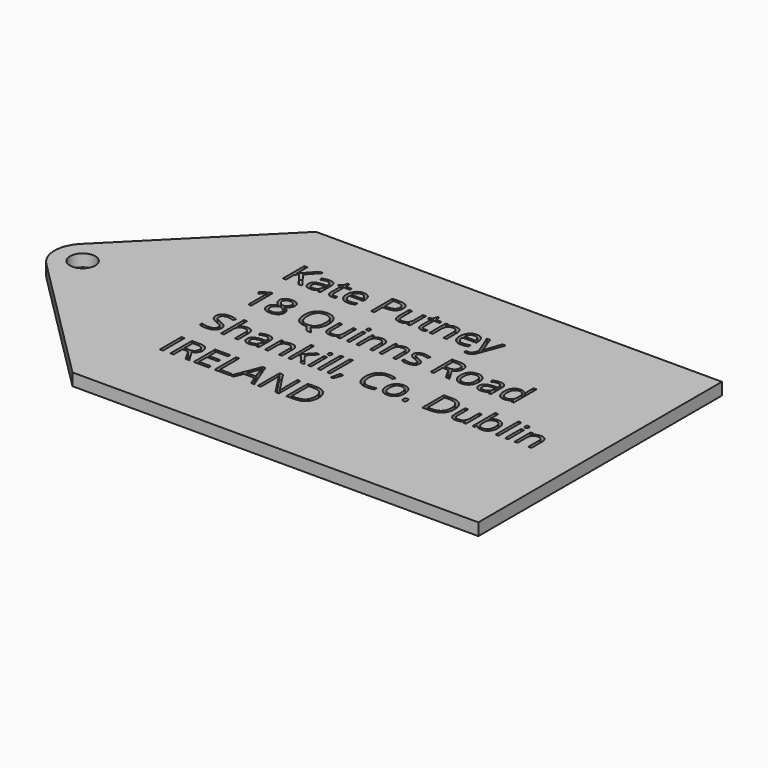
from build123d import *

# Parameters (mm, degrees)
F0_R         = 2.5
F0_W         = 80
F0_H         = 60
F1_DEPTH     = 2.4
F2_TEXT_SIZE = 7.4209044227
F3_DEPTH     = 1.2


# Not quite as in the source:
# - Text() gives the source's letters only with a copy of the font that has no kerning and outlines rounded to 1/6400 em; it was checked with that copy


with BuildPart() as f1:
    # F0 (on Top) → F1 (new body)
    with BuildSketch(Plane.XY):
        with BuildLine():
            Line((-23.865801543, -30), (-23.865801543, 30))
            Line((-23.865801543, 30), (-49.6231608559, 4.2426406871))
            ThreePointArc((-49.6231608559, 4.2426406871), (-51.3805201688, 0), (-49.6231608559, -4.2426406871))
            Line((-49.6231608559, -4.2426406871), (-23.865801543, -30))
        make_face()
        with Locations((-45.865801543, 0)):
            Circle(F0_R, mode=Mode.SUBTRACT)
        with Locations((16.134198457, 0)):
            Rectangle(F0_W, F0_H)
    extrude(amount=F1_DEPTH)

    # F2 (on face) → F3 (cut)
    with BuildSketch(Plane.XY.offset(2.4)):
        with Locations((-18.865801543, 14.6569488156)):
            Text('Kate Putney', F2_TEXT_SIZE, font='Open Sans', text_align=(TextAlign.LEFT, TextAlign.BOTTOM))
        with Locations((-18.865801543, 4.5645188007)):
            Text('18 Quinns Road', F2_TEXT_SIZE, font='Open Sans', text_align=(TextAlign.LEFT, TextAlign.BOTTOM))
        with Locations((-18.865801543, -5.5279112142)):
            Text('Shankill, Co. Dublin', F2_TEXT_SIZE, font='Open Sans', text_align=(TextAlign.LEFT, TextAlign.BOTTOM))
        with Locations((-18.865801543, -15.6203412291)):
            Text('IRELAND', F2_TEXT_SIZE, font='Open Sans', text_align=(TextAlign.LEFT, TextAlign.BOTTOM))
    extrude(amount=-F3_DEPTH, mode=Mode.SUBTRACT)


solid = f1.part
